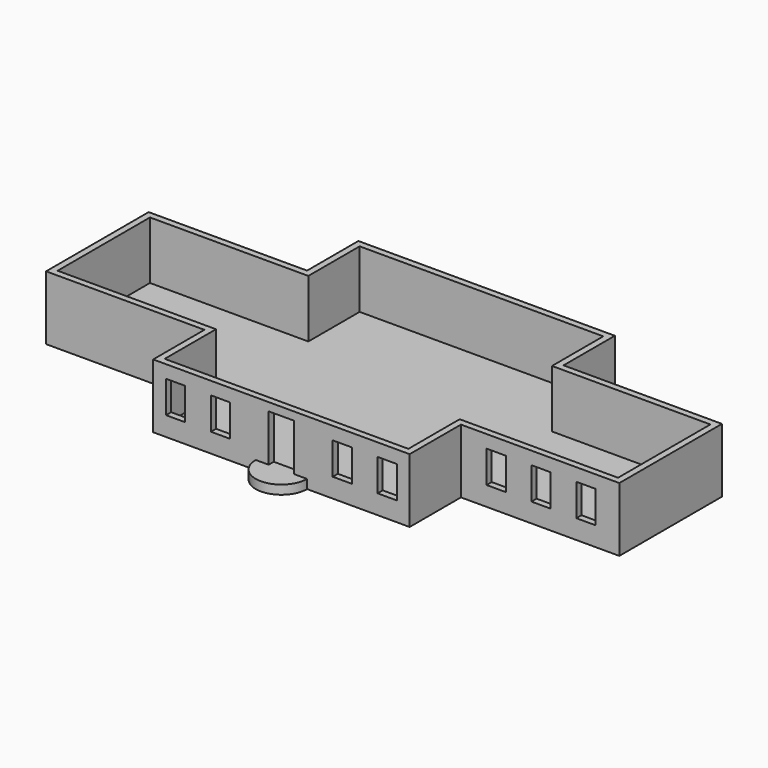
from build123d import *

# Parameters (mm, degrees)
F1_DEPTH = 10
F2_T     = -1
F3_DEPTH = 1.4
F4_W     = 3
F4_H     = 5
F4_W_2   = 3.991
F4_H_2   = 7.333
F5_DEPTH = 12


with BuildPart() as f1:
    # F0 (on Top) → F1 (new body)
    with BuildSketch(Plane.XY):
        with BuildLine():
            Line((-44.662655282, 31.9538097456), (-44.662655282, 21.9538097456))
            Line((-44.662655282, 21.9538097456), (-69.362655282, 21.9538097456))
            Line((-69.362655282, 21.9538097456), (-69.362655282, 1.9538097456))
            Line((-69.362655282, 1.9538097456), (-44.662655282, 1.9538097456))
            Line((-44.662655282, 1.9538097456), (-44.662655282, -8.0461902544))
            Line((-44.662655282, -8.0461902544), (-28.662655282, -8.0461902544))
            ThreePointArc((-28.662655282, -8.0461902544), (-24.662655282, -4.0461902544), (-20.662655282, -8.0461902544))
            Line((-20.662655282, -8.0461902544), (-4.662655282, -8.0461902544))
            Line((-4.662655282, -8.0461902544), (-4.662655282, 1.9538097456))
            Line((-4.662655282, 1.9538097456), (20.037344718, 1.9538097456))
            Line((20.037344718, 1.9538097456), (20.037344718, 21.9538097456))
            Line((20.037344718, 21.9538097456), (-4.662655282, 21.9538097456))
            Line((-4.662655282, 21.9538097456), (-4.662655282, 31.9538097456))
            Line((-4.662655282, 31.9538097456), (-44.662655282, 31.9538097456))
        make_face()
        with BuildLine():
            ThreePointArc((-20.662655282, -8.0461902544), (-24.662655282, -4.0461902544), (-28.662655282, -8.0461902544))
            Line((-28.662655282, -8.0461902544), (-20.662655282, -8.0461902544))
        make_face()
    extrude(amount=F1_DEPTH)

    # F2
    f2_openings = [f1.faces().sort_by_distance(p)[0] for p in [
        (-24.662655, 11.95381, 10),
    ]]
    offset(amount=F2_T, openings=f2_openings, kind=Kind.INTERSECTION)

    # F0 (on Top) → F3 (join)
    with BuildSketch(Plane.XY):
        with BuildLine():
            Line((-20.662655282, -8.0461902544), (-28.662655282, -8.0461902544))
            ThreePointArc((-28.662655282, -8.0461902544), (-24.662655282, -12.0461902544), (-20.662655282, -8.0461902544))
        make_face()
    extrude(amount=F3_DEPTH)

    # F4 (on face) → F5 (cut)
    with BuildSketch(Plane.XZ.offset(8.0461902544)):
        with Locations((-41.162655282, 5.5)):
            Rectangle(F4_W, F4_H)
        with Locations((-34.162655282, 5.5)):
            Rectangle(F4_W, F4_H)
        with Locations((-15.162655282, 5.5)):
            Rectangle(F4_W, F4_H)
        with Locations((-8.162655282, 5.5)):
            Rectangle(F4_W, F4_H)
        with Locations((0.837344718, 5.5)):
            Rectangle(F4_W, F4_H)
        with Locations((7.837344718, 5.5)):
            Rectangle(F4_W, F4_H)
        with Locations((14.837344718, 5.5)):
            Rectangle(F4_W, F4_H)
        with Locations((-24.658155282, 5.0665)):
            Rectangle(F4_W_2, F4_H_2)
    extrude(amount=-F5_DEPTH, mode=Mode.SUBTRACT)


solid = f1.part
